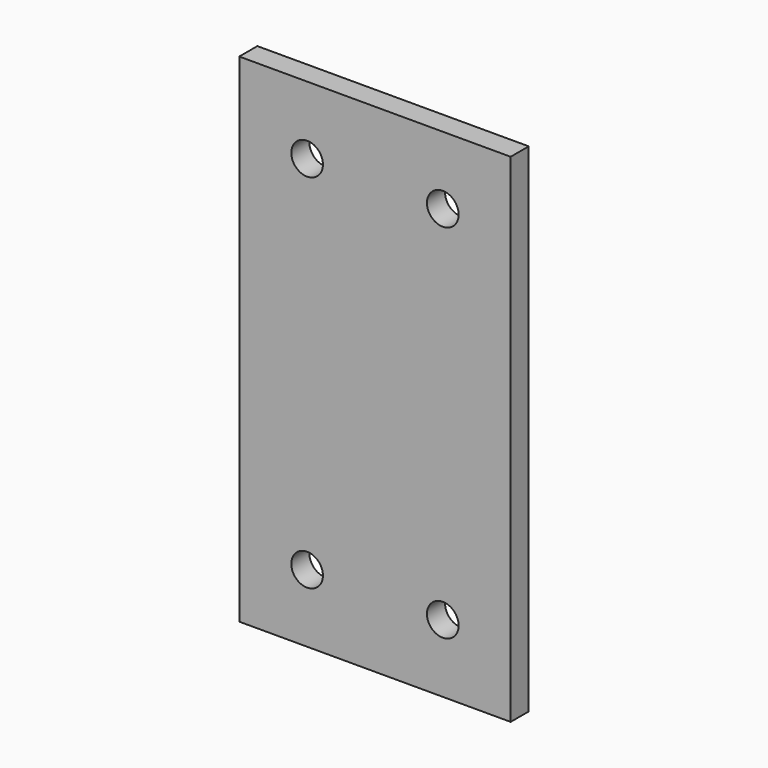
from build123d import *

# Parameters (mm, degrees)
F0_W     = 120
F0_H     = 220
F0_R     = 7
F1_DEPTH = 10


# Not quite as in the source:
# - a feature names something its author has since deleted; it is built from what else it names


with BuildPart() as f1:
    # F0 (on Front) → F1 (new body)
    with BuildSketch(Plane.XZ):
        Rectangle(F0_W, F0_H)
        with Locations((-30, -80)):
            Circle(F0_R, mode=Mode.SUBTRACT)
        with Locations((30, -80)):
            Circle(F0_R, mode=Mode.SUBTRACT)
        with Locations((-30, 80)):
            Circle(F0_R, mode=Mode.SUBTRACT)
        with Locations((30, 80)):
            Circle(F0_R, mode=Mode.SUBTRACT)
    extrude(amount=F1_DEPTH)


solid = f1.part
